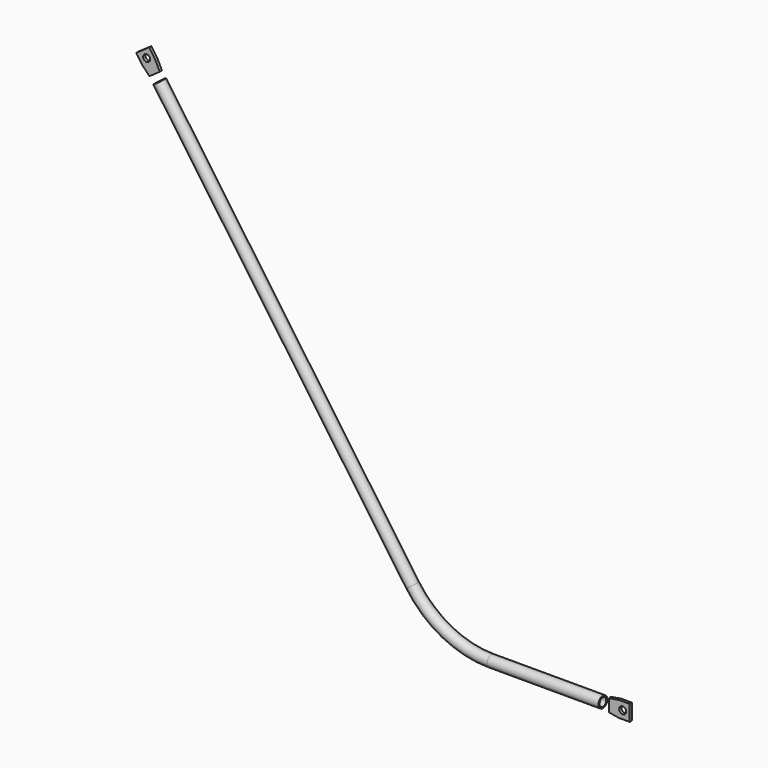
from build123d import *

# Parameters (mm, degrees)
F1_R      = 4
F1_R_2    = 3
F3_W      = 40
F3_H      = 27.601965531
F4_DEPTH  = 12.5
F6_DEPTH  = 1
F9_R      = 2.5
F10_DEPTH = 5.0010001


# Not quite as in the source:
# - the program builds the solid bodies; features that only make, move or delete a surface that nothing else refers to are left out


with BuildPart() as f2:
    # F2: sweep along a path in F0
    with BuildLine(Plane.XZ) as f2_path:
        Line((0, 0), (-100, 0))
        ThreePointArc((-100, 0), (-131.9137554037, 7.8092462649), (-156.615693541, 29.4722646016))
        Line((-156.615693541, 29.4722646016), (-349.6815220168, 305.1988427093))
    # F1 (on Right) → F2 (sweep)
    with BuildSketch(Plane.YZ):
        Circle(F1_R)
        Circle(F1_R_2, mode=Mode.SUBTRACT)
    sweep(path=f2_path.line)

    # F3 (on Front) → F4 (cut, symmetric)
    with BuildSketch(Plane.XZ):
        Rectangle(F3_W, F3_H)
        Polygon((-346.4049138396, 307.4931484547), (-352.958130194, 302.9045369639), (-341.4866014669, 286.5214960781), (-334.9333851126, 291.1101075689), align=None)
    extrude(amount=F4_DEPTH, both=True, mode=Mode.SUBTRACT)


with BuildPart() as f6:
    # F5 (on Front) → F6 (new body, symmetric)
    with BuildSketch(Plane.XZ):
        Polygon((0, -5.7), (0, 5.7), (-7.5, 5.7), (-15, 4.5), (-15, -4.5), (-7.5, -5.7), align=None)
    extrude(amount=F6_DEPTH, both=True)


with BuildPart() as f6b:
    # F5 (on Front) → F6, piece 2 (new body, symmetric)
    with BuildSketch(Plane.XZ):
        Polygon((-345.0123553643, 308.4682283965), (-354.3506886692, 301.9294570221), (-350.0488653966, 295.7858166899), (-344.7640596708, 290.3304680814), (-337.3916912722, 295.4926560085), (-340.7105320917, 302.3245880643), align=None)
    extrude(amount=F6_DEPTH, both=True)


with BuildPart() as f10_tool:
    # F9 (on face) → F10 (new body, through all)
    with BuildSketch(Plane.XZ.offset(1)):
        with Locations((-346.813639835, 301.1030824878)):
            Circle(F9_R)
        with Locations((-5, 0)):
            Circle(F9_R)
    extrude(amount=-F10_DEPTH)


with BuildPart() as f6_1:
    add(f6.part)

    # F10: cut by f10_tool
    add(f10_tool.part, mode=Mode.SUBTRACT)


with BuildPart() as f6b_1:
    add(f6b.part)

    # F10: cut by f10_tool
    add(f10_tool.part, mode=Mode.SUBTRACT)


solid = Compound([f2.part, f6_1.part, f6b_1.part])
